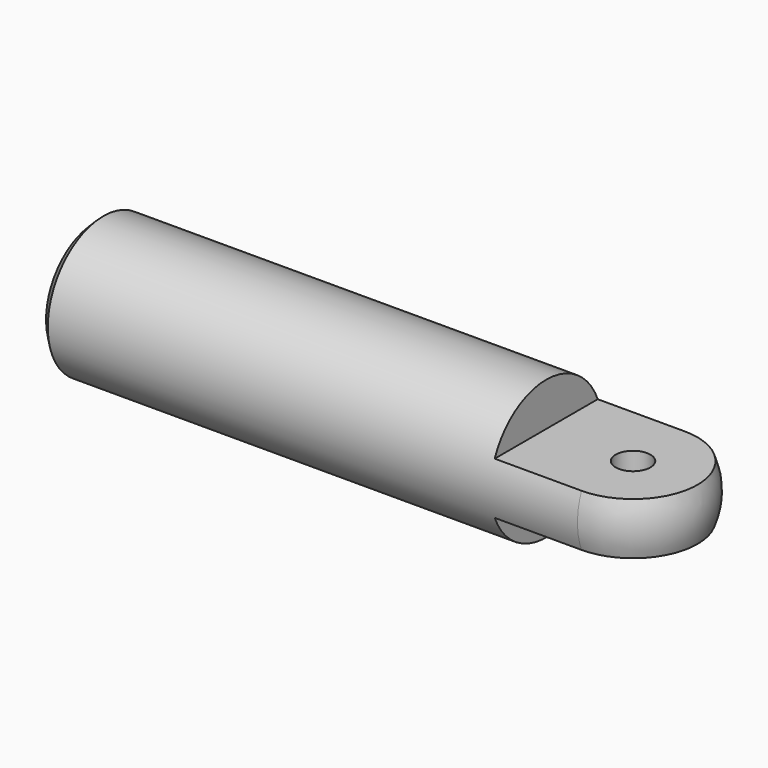
from build123d import *

# Parameters (mm, degrees)
F2_SIZE  = 0.5
F4_START = -1.5
F4_DEPTH = 6.5
F5_R     = 1
F6_DEPTH = 1.5


# Not quite as in the source:
# - a pattern or mirror of a feature is missing from the dataset's text; its kind, count and spacing are read off the source's solid


with BuildPart() as f1:
    # F0 (on Front) → F1 (revolve)
    with BuildSketch(Plane.XZ):
        with BuildLine():
            Line((0, 4), (0, 0))
            Line((0, 0), (35, 0))
            ThreePointArc((35, 0), (33.8284271247, 2.8284271247), (31, 4))
            Line((31, 4), (0, 4))
        make_face()
    revolve(axis=Axis((22.9748431593, 0, 0), (1, 0, 0)))

    # F2
    f2_edges = [f1.edges().sort_by_distance(p)[0] for p in [
        (0, 0, -4),
    ]]
    chamfer(f2_edges, length=F2_SIZE)

    # F3 (on Top) → F4 (cut)
    with BuildSketch(Plane.XY.offset(F4_START)):
        with BuildLine():
            Line((26, -4), (31, -4))
            ThreePointArc((31, -4), (35, 0), (31, 4))
            Line((31, 4), (26, 4))
            Line((26, 4), (26, -4))
        make_face()
    f4 = extrude(amount=-F4_DEPTH, mode=Mode.SUBTRACT)

    # F4_copies: F4 across plane
    add(f4.mirror(Plane.XY), mode=Mode.SUBTRACT)

    # F5 (on Top) → F6 (cut, symmetric)
    with BuildSketch(Plane.XY):
        with Locations((31, 0)):
            Circle(F5_R)
    extrude(amount=F6_DEPTH, both=True, mode=Mode.SUBTRACT)


solid = f1.part
